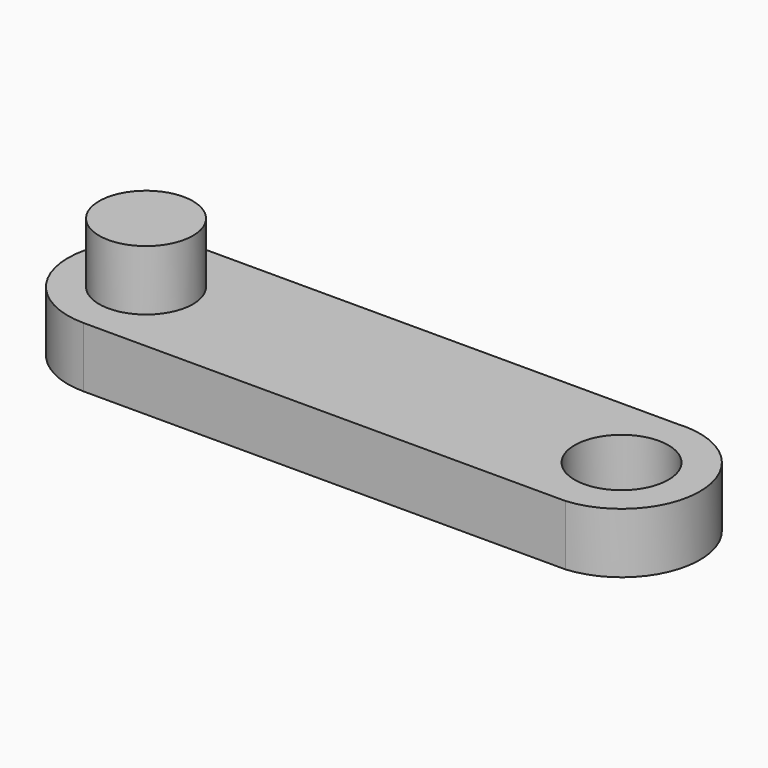
from build123d import *

# Parameters (mm, degrees)
F2_DEPTH = 12.7
F3_R     = 9.8806
F4_DEPTH = 12.7
F5_DEPTH = 12.7


# Not quite as in the source:
# - a variable given as a bare number and used for a length is read in inches; the dataset says mm whatever the document's units were


with BuildPart() as f2:
    # F1 (on Top) → F2 (new body)
    with BuildSketch(Plane.XY):
        with BuildLine():
            ThreePointArc((50.8, -16.9333333333), (65.8706666667, 0.9313333333), (48.006, 16.002))
            Line((48.006, 16.002), (-50.8, 16.002))
            ThreePointArc((-50.8, 16.002), (-67.2676666667, -0.4656666667), (-50.8, -16.9333333333))
            Line((-50.8, -16.9333333333), (50.8, -16.9333333333))
        make_face()
    extrude(amount=F2_DEPTH)

    # F3 (on face) → F4 (join)
    with BuildSketch(Plane.XY.offset(12.7)):
        with Locations((-50.8, -0.4656666667)):
            Circle(F3_R)
    extrude(amount=F4_DEPTH)

    # F3 (on face) → F5 (cut)
    with BuildSketch(Plane.XY.offset(12.7)):
        with Locations((49.403, -0.4656666667)):
            Circle(F3_R)
    extrude(amount=-F5_DEPTH, mode=Mode.SUBTRACT)


solid = f2.part
